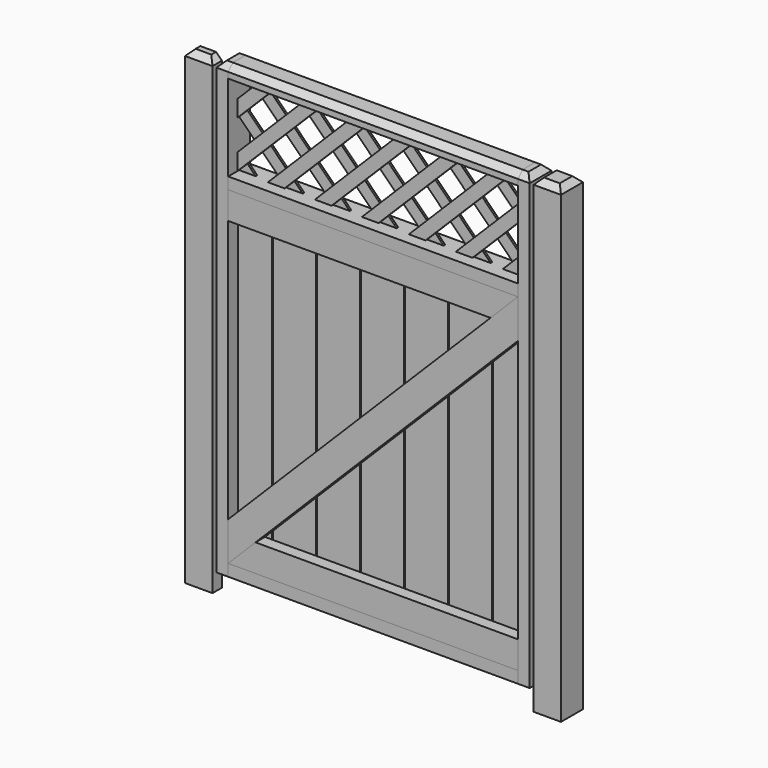
from build123d import *

# Parameters (mm, degrees)
F0_W       = 88.9
F0_H       = 88.9
F1_DEPTH   = 1524
F0_H_2     = 38.1
F3_DEPTH   = 88.9
F4_W       = 939.8
F4_H       = 38.1
F5_DEPTH   = 88.9
F7_DEPTH   = 38.1
F9_DEPTH   = 38.1
F10_W      = 139.7
F10_H      = 1066.8
F11_DEPTH  = 15.875
F10_W_2    = 109.5375
F12_W      = 939.8
F12_H      = 88.9
F13_DEPTH  = 15.875
F16_DEPTH  = 6.35
F18_DEPTH  = 6.35
F19_SIZE   = 19.05
F19_2_SIZE = 19.05
F19_3_SIZE = 19.05
F19_4_SIZE = 19.05
F19_5_SIZE = 19.05


with BuildPart() as f1:
    # F0 (on Top) → F1 (new body)
    with BuildSketch(Plane.XY):
        with Locations((1085.85, 44.45)):
            Rectangle(F0_W, F0_H)
    extrude(amount=F1_DEPTH)

    # F19
    f19_edges = [f1.edges().sort_by_distance(p)[0] for p in [
        (1041.4, 44.45, 1524),
        (1085.85, 0, 1524),
        (1130.3, 44.45, 1524),
        (1085.85, 88.9, 1524),
    ]]
    chamfer(f19_edges, length=F19_SIZE)


with BuildPart() as f1b:
    # F0 (on Top) → F1, piece 2 (new body)
    with BuildSketch(Plane.XY):
        with Locations((-44.45, 19.05)):
            Rectangle(F0_W, F0_H_2)
    extrude(amount=F1_DEPTH)

    # F19#2
    f19_2_edges = [f1b.edges().sort_by_distance(p)[0] for p in [
        (-44.45, 0, 1524),
        (0, 19.05, 1524),
        (-88.9, 19.05, 1524),
    ]]
    chamfer(f19_2_edges, length=F19_2_SIZE)


with BuildPart() as f3:
    # F2 (on face) → F3 (new body)
    with BuildSketch(Plane.XZ):
        Polygon((1028.7, 63.5), (1028.7, 1524), (990.6, 1524), (990.6, 1485.9), (990.6, 1206.5), (990.6, 1168.4), (990.6, 101.6), (990.6, 63.5), align=None)
    extrude(amount=-F3_DEPTH)

    # F19#3
    f19_3_edges = [f3.edges().sort_by_distance(p)[0] for p in [
        (1009.65, 0, 1524),
        (1028.7, 44.45, 1524),
        (1009.65, 88.9, 1524),
    ]]
    chamfer(f19_3_edges, length=F19_3_SIZE)


with BuildPart() as f3b:
    # F2 (on face) → F3, piece 2 (new body)
    with BuildSketch(Plane.XZ):
        Polygon((50.8, 1485.9), (50.8, 1524), (12.7, 1524), (12.7, 63.5), (50.8, 63.5), (50.8, 101.6), (50.8, 1168.4), (50.8, 1206.5), align=None)
    extrude(amount=-F3_DEPTH)

    # F19#4
    f19_4_edges = [f3b.edges().sort_by_distance(p)[0] for p in [
        (31.75, 0, 1524),
        (12.7, 44.45, 1524),
        (31.75, 88.9, 1524),
    ]]
    chamfer(f19_4_edges, length=F19_4_SIZE)


with BuildPart() as f5:
    # F4 (on face) → F5 (new body)
    with BuildSketch(Plane.XZ):
        with Locations((520.7, 1504.95)):
            Rectangle(F4_W, F4_H)
    extrude(amount=-F5_DEPTH)

    # F19#5
    f19_5_edges = [f5.edges().sort_by_distance(p)[0] for p in [
        (520.7, 0, 1524),
        (520.7, 88.9, 1524),
    ]]
    chamfer(f19_5_edges, length=F19_5_SIZE)


with BuildPart() as f5b:
    # F4 (on face) → F5, piece 2 (new body)
    with BuildSketch(Plane.XZ):
        with Locations((520.7, 1187.45)):
            Rectangle(F4_W, F4_H)
    extrude(amount=-F5_DEPTH)


with BuildPart() as f5c:
    # F4 (on face) → F5, piece 3 (new body)
    with BuildSketch(Plane.XZ):
        with Locations((520.7, 82.55)):
            Rectangle(F4_W, F4_H)
    extrude(amount=-F5_DEPTH)


with BuildPart() as f7:
    # F6 (on face) → F7 (new body)
    with BuildSketch(Plane.XZ):
        Polygon((990.6, 1042.596365767), (990.6, 1168.4), (50.8, 227.403634233), (50.8, 101.6), align=None)
    extrude(amount=-F7_DEPTH)


with BuildPart() as f9:
    # F8 (on face) → F9 (new body)
    with BuildSketch(Plane.XZ):
        Polygon((990.6, 1168.4), (50.8, 1168.4), (50.8, 1079.5), (901.8130258528, 1079.5), align=None)
    extrude(amount=-F9_DEPTH)


with BuildPart() as f9b:
    # F8 (on face) → F9, piece 2 (new body)
    with BuildSketch(Plane.XZ):
        Polygon((50.8, 101.6), (990.6, 101.6), (990.6, 190.5), (139.5869741472, 190.5), align=None)
    extrude(amount=-F9_DEPTH)


with BuildPart() as f11:
    # F10 (on face) → F11 (new body)
    with BuildSketch(Plane(origin=(0, 38.1, 0), x_dir=(-1, 0, 0), z_dir=(0, 1, 0))):
        with Locations((-520.7, 635)):
            Rectangle(F10_W, F10_H)
    extrude(amount=F11_DEPTH)


with BuildPart() as f11b:
    # F10 (on face) → F11, piece 2 (new body)
    with BuildSketch(Plane(origin=(0, 38.1, 0), x_dir=(-1, 0, 0), z_dir=(0, 1, 0))):
        with Locations((-377.825, 635)):
            Rectangle(F10_W, F10_H)
    extrude(amount=F11_DEPTH)


with BuildPart() as f11c:
    # F10 (on face) → F11, piece 3 (new body)
    with BuildSketch(Plane(origin=(0, 38.1, 0), x_dir=(-1, 0, 0), z_dir=(0, 1, 0))):
        with Locations((-234.95, 635)):
            Rectangle(F10_W, F10_H)
    extrude(amount=F11_DEPTH)


with BuildPart() as f11d:
    # F10 (on face) → F11, piece 4 (new body)
    with BuildSketch(Plane(origin=(0, 38.1, 0), x_dir=(-1, 0, 0), z_dir=(0, 1, 0))):
        with Locations((-107.15625, 635)):
            Rectangle(F10_W_2, F10_H)
    extrude(amount=F11_DEPTH)


with BuildPart() as f11e:
    # F10 (on face) → F11, piece 5 (new body)
    with BuildSketch(Plane(origin=(0, 38.1, 0), x_dir=(-1, 0, 0), z_dir=(0, 1, 0))):
        with Locations((-806.45, 635)):
            Rectangle(F10_W, F10_H)
    extrude(amount=F11_DEPTH)


with BuildPart() as f11f:
    # F10 (on face) → F11, piece 6 (new body)
    with BuildSketch(Plane(origin=(0, 38.1, 0), x_dir=(-1, 0, 0), z_dir=(0, 1, 0))):
        with Locations((-934.24375, 635)):
            Rectangle(F10_W_2, F10_H)
    extrude(amount=F11_DEPTH)


with BuildPart() as f11g:
    # F10 (on face) → F11, piece 7 (new body)
    with BuildSketch(Plane(origin=(0, 38.1, 0), x_dir=(-1, 0, 0), z_dir=(0, 1, 0))):
        with Locations((-663.575, 635)):
            Rectangle(F10_W, F10_H)
    extrude(amount=F11_DEPTH)


with BuildPart() as f13:
    # F12 (on face) → F13 (new body)
    with BuildSketch(Plane(origin=(0, 53.975, 0), x_dir=(-1, 0, 0), z_dir=(0, 1, 0))):
        with Locations((-520.7, 1123.95)):
            Rectangle(F12_W, F12_H)
    extrude(amount=F13_DEPTH)


with BuildPart() as f13b:
    # F12 (on face) → F13, piece 2 (new body)
    with BuildSketch(Plane(origin=(0, 53.975, 0), x_dir=(-1, 0, 0), z_dir=(0, 1, 0))):
        with Locations((-520.7, 146.05)):
            Rectangle(F12_W, F12_H)
    extrude(amount=F13_DEPTH)


with BuildPart() as f16:
    # F15 (on offset) → F16 (new body)
    with BuildSketch(Plane.XZ.offset(-44.45)):
        Polygon((177.8, 1485.9), (123.9184632736, 1485.9), (50.8, 1412.7815367264), (50.8, 1358.9), align=None)
    extrude(amount=F16_DEPTH)


with BuildPart() as f16b:
    # F15 (on offset) → F16, piece 2 (new body)
    with BuildSketch(Plane.XZ.offset(-44.45)):
        Polygon((990.6, 1384.3), (990.6, 1438.1815367264), (758.9184632736, 1206.5), (812.8, 1206.5), align=None)
    extrude(amount=F16_DEPTH)


with BuildPart() as f16c:
    # F15 (on offset) → F16, piece 3 (new body)
    with BuildSketch(Plane.XZ.offset(-44.45)):
        Polygon((50.8, 1260.3815367264), (50.8, 1206.5), (330.2, 1485.9), (276.3184632736, 1485.9), align=None)
    extrude(amount=F16_DEPTH)


with BuildPart() as f16d:
    # F15 (on offset) → F16, piece 4 (new body)
    with BuildSketch(Plane.XZ.offset(-44.45)):
        Polygon((149.3184632736, 1206.5), (203.2, 1206.5), (482.6, 1485.9), (428.7184632736, 1485.9), align=None)
    extrude(amount=F16_DEPTH)


with BuildPart() as f16e:
    # F15 (on offset) → F16, piece 5 (new body)
    with BuildSketch(Plane.XZ.offset(-44.45)):
        Polygon((301.7184632736, 1206.5), (355.6, 1206.5), (635, 1485.9), (581.1184632736, 1485.9), align=None)
    extrude(amount=F16_DEPTH)


with BuildPart() as f16f:
    # F15 (on offset) → F16, piece 6 (new body)
    with BuildSketch(Plane.XZ.offset(-44.45)):
        Polygon((454.1184632736, 1206.5), (508, 1206.5), (787.4, 1485.9), (733.5184632736, 1485.9), align=None)
    extrude(amount=F16_DEPTH)


with BuildPart() as f16g:
    # F15 (on offset) → F16, piece 7 (new body)
    with BuildSketch(Plane.XZ.offset(-44.45)):
        Polygon((606.5184632736, 1206.5), (660.4, 1206.5), (939.8, 1485.9), (885.9184632736, 1485.9), align=None)
    extrude(amount=F16_DEPTH)


with BuildPart() as f16h:
    # F15 (on offset) → F16, piece 8 (new body)
    with BuildSketch(Plane.XZ.offset(-44.45)):
        Polygon((911.3184632736, 1206.5), (965.2, 1206.5), (990.6, 1231.9), (990.6, 1285.7815367264), align=None)
    extrude(amount=F16_DEPTH)


with BuildPart() as f18:
    # F17 (on offset) → F18 (new body)
    with BuildSketch(Plane.XZ.offset(-44.45)):
        Polygon((104.6815367264, 1206.5), (50.8, 1260.3815367264), (50.8, 1206.5), align=None)
    extrude(amount=-F18_DEPTH)


with BuildPart() as f18b:
    # F17 (on offset) → F18, piece 2 (new body)
    with BuildSketch(Plane.XZ.offset(-44.45)):
        Polygon((257.0815367264, 1206.5), (50.8, 1412.7815367264), (50.8, 1358.9), (203.2, 1206.5), align=None)
    extrude(amount=-F18_DEPTH)


with BuildPart() as f18c:
    # F17 (on offset) → F18, piece 3 (new body)
    with BuildSketch(Plane.XZ.offset(-44.45)):
        Polygon((409.4815367264, 1206.5), (130.0815367264, 1485.9), (76.2, 1485.9), (355.6, 1206.5), align=None)
    extrude(amount=-F18_DEPTH)


with BuildPart() as f18d:
    # F17 (on offset) → F18, piece 4 (new body)
    with BuildSketch(Plane.XZ.offset(-44.45)):
        Polygon((561.8815367264, 1206.5), (282.4815367264, 1485.9), (228.6, 1485.9), (508, 1206.5), align=None)
    extrude(amount=-F18_DEPTH)


with BuildPart() as f18e:
    # F17 (on offset) → F18, piece 5 (new body)
    with BuildSketch(Plane.XZ.offset(-44.45)):
        Polygon((714.2815367264, 1206.5), (434.8815367264, 1485.9), (381, 1485.9), (660.4, 1206.5), align=None)
    extrude(amount=-F18_DEPTH)


with BuildPart() as f18f:
    # F17 (on offset) → F18, piece 6 (new body)
    with BuildSketch(Plane.XZ.offset(-44.45)):
        Polygon((866.6815367264, 1206.5), (587.2815367264, 1485.9), (533.4, 1485.9), (812.8, 1206.5), align=None)
    extrude(amount=-F18_DEPTH)


with BuildPart() as f18g:
    # F17 (on offset) → F18, piece 7 (new body)
    with BuildSketch(Plane.XZ.offset(-44.45)):
        Polygon((990.6, 1234.9815367264), (739.6815367264, 1485.9), (685.8, 1485.9), (965.2, 1206.5), (990.6, 1206.5), align=None)
    extrude(amount=-F18_DEPTH)


with BuildPart() as f18h:
    # F17 (on offset) → F18, piece 8 (new body)
    with BuildSketch(Plane.XZ.offset(-44.45)):
        Polygon((990.6, 1387.3815367264), (892.0815367264, 1485.9), (838.2, 1485.9), (990.6, 1333.5), align=None)
    extrude(amount=-F18_DEPTH)


solid = Compound([f1.part, f1b.part, f3.part, f3b.part, f5.part, f5b.part, f5c.part, f7.part, f9.part, f9b.part, f11.part, f11b.part, f11c.part, f11d.part, f11e.part, f11f.part, f11g.part, f13.part, f13b.part, f16.part, f16b.part, f16c.part, f16d.part, f16e.part, f16f.part, f16g.part, f16h.part, f18.part, f18b.part, f18c.part, f18d.part, f18e.part, f18f.part, f18g.part, f18h.part])
